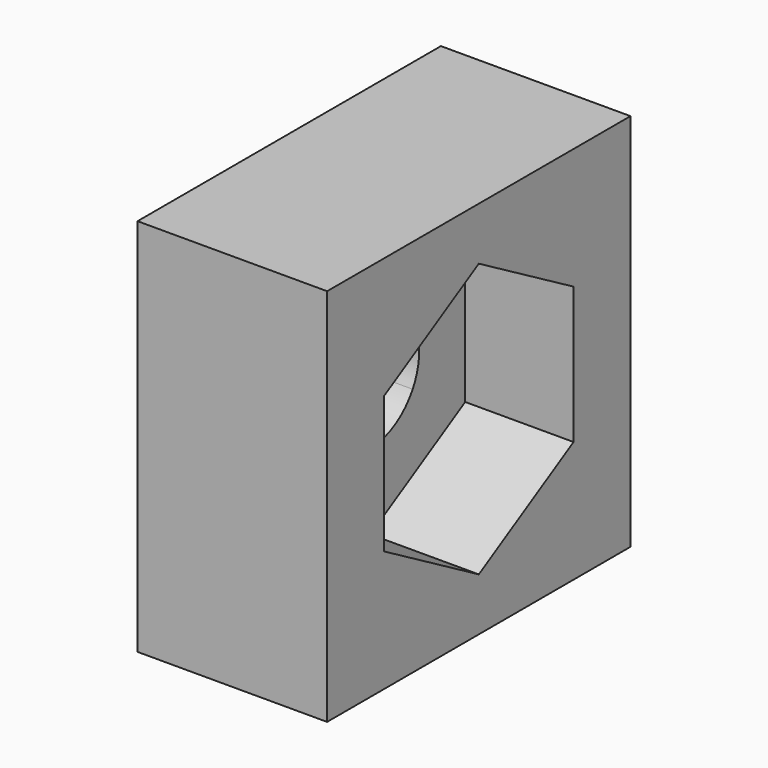
from build123d import *

# Parameters (mm, degrees)
F0_W     = 14
F0_H     = 14
F1_DEPTH = 3
F2_W     = 14
F2_H     = 14
F3_DEPTH = 4
F4_ANGLE = -90
F5_ANGLE = -90


# Not quite as in the source:
# - a feature names something its author has since deleted; it is built from what else it names


with BuildPart() as f1:
    # F0 (on Top) → F1 (new body)
    with BuildSketch(Plane.XY):
        Rectangle(F0_W, F0_H)
        with BuildLine():
            ThreePointArc((1.9485571585, 1.125), (2.1733331092, 0.5823428515), (2.25, 0))
            ThreePointArc((2.25, 0), (2.1733331092, -0.5823428515), (1.9485571585, -1.125))
            ThreePointArc((1.9485571585, -1.125), (-2.25, 0), (1.9485571585, 1.125))
        make_face(mode=Mode.SUBTRACT)
    extrude(amount=F1_DEPTH)

    # F2 (on face) → F3 (join)
    with BuildSketch(Plane.XY.offset(3)):
        Rectangle(F2_W, F2_H)
        with BuildLine():
            ThreePointArc((4.3734282891, 2.525), (4.8779254228, 1.3070361778), (5.05, 0))
            ThreePointArc((5.05, 0), (4.8779254228, -1.3070361778), (4.3734282891, -2.525))
            ThreePointArc((4.3734282891, -2.525), (2.525, -4.3734282891), (0, -5.05))
            ThreePointArc((0, -5.05), (-2.525, -4.3734282891), (-4.3734282891, -2.525))
            ThreePointArc((-4.3734282891, -2.525), (-5.05, 0), (-4.3734282891, 2.525))
            ThreePointArc((-4.3734282891, 2.525), (-2.525, 4.3734282891), (0, 5.05))
            ThreePointArc((0, 5.05), (2.525, 4.3734282891), (4.3734282891, 2.525))
        make_face(mode=Mode.SUBTRACT)
        with BuildLine():
            Line((-4.3734282891, -2.525), (-4.3734282891, 2.525))
            ThreePointArc((-4.3734282891, 2.525), (-5.05, 0), (-4.3734282891, -2.525))
        make_face()
        with BuildLine():
            Line((-4.3734282891, 2.525), (0, 5.05))
            ThreePointArc((0, 5.05), (-2.525, 4.3734282891), (-4.3734282891, 2.525))
        make_face()
        with BuildLine():
            Line((0, 5.05), (4.3734282891, 2.525))
            ThreePointArc((4.3734282891, 2.525), (2.525, 4.3734282891), (0, 5.05))
        make_face()
        with BuildLine():
            ThreePointArc((4.3734282891, -2.525), (4.8779254228, -1.3070361778), (5.05, 0))
            ThreePointArc((5.05, 0), (4.8779254228, 1.3070361778), (4.3734282891, 2.525))
            Line((4.3734282891, 2.525), (4.3734282891, -2.525))
        make_face()
        with BuildLine():
            ThreePointArc((0, -5.05), (2.525, -4.3734282891), (4.3734282891, -2.525))
            Line((4.3734282891, -2.525), (0, -5.05))
        make_face()
        with BuildLine():
            ThreePointArc((-4.3734282891, -2.525), (-2.525, -4.3734282891), (0, -5.05))
            Line((0, -5.05), (-4.3734282891, -2.525))
        make_face()
    extrude(amount=F3_DEPTH)


with BuildPart() as f1_1:
    # F4: moved
    add(f1.part.rotate(Axis((0, -7, 0), (-1, 0, 0)), F4_ANGLE))


with BuildPart() as f1_2:
    # F5: moved
    add(f1_1.part.rotate(Axis((7, -7, 7), (0, 0, -1)), F5_ANGLE))


solid = f1_2.part
